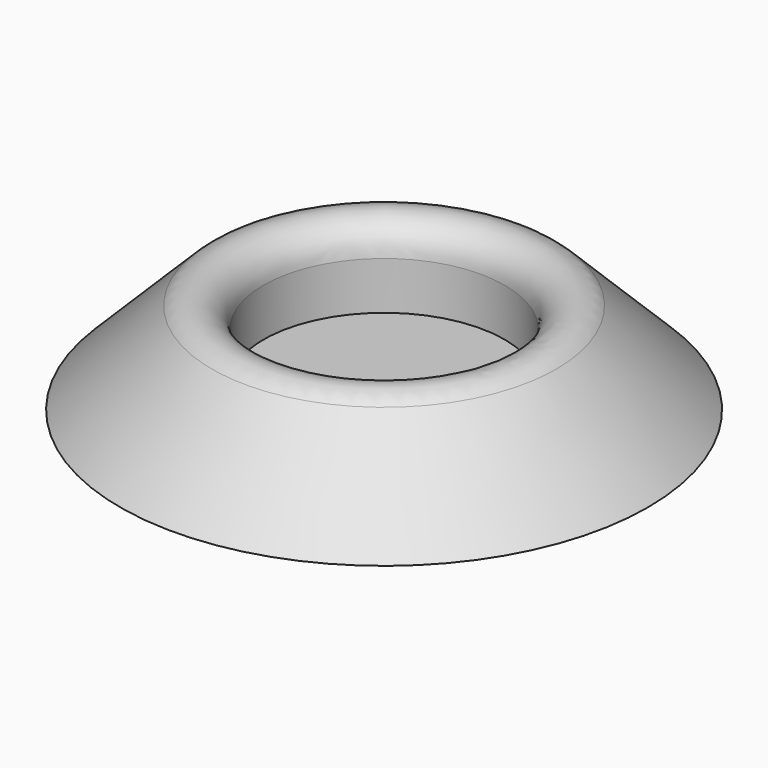
from build123d import *

# Parameters (mm, degrees)
F0_R     = 17.5
F1_DEPTH = 10
F2_R     = 8
F3_DEPTH = 8.5
F5_R     = 2


# Not quite as in the source:
# - a fillet or chamfer that OpenCascade refuses, or shapes differently, is made with other operations: its cross-section is extruded or revolved along the edge and cut away or added


with BuildPart() as f1:
    # F0 (on Top) → F1 (new body)
    with BuildSketch(Plane.XY):
        Circle(F0_R)
    extrude(amount=F1_DEPTH)

    # F2 (on face) → F3 (cut)
    with BuildSketch(Plane.XY.offset(10)):
        Circle(F2_R)
    extrude(amount=-F3_DEPTH, mode=Mode.SUBTRACT)

    # F4: chamfer of 10 on 1 edges, made by hand

    # F4_s1 → F4_t2 (revolve, cut)
    with BuildSketch(Plane.XZ):
        Polygon((17.5, 0), (7.5, 10), (17.5, 10), align=None)
    revolve(axis=Axis((0, 0, 10), (0, 0, 1)), mode=Mode.SUBTRACT)

    # F5
    f5_edges = [f1.edges().sort_by_distance(p)[0] for p in [
        (-8, 0, 9.5),
    ]]
    fillet(f5_edges, radius=F5_R)


solid = f1.part
